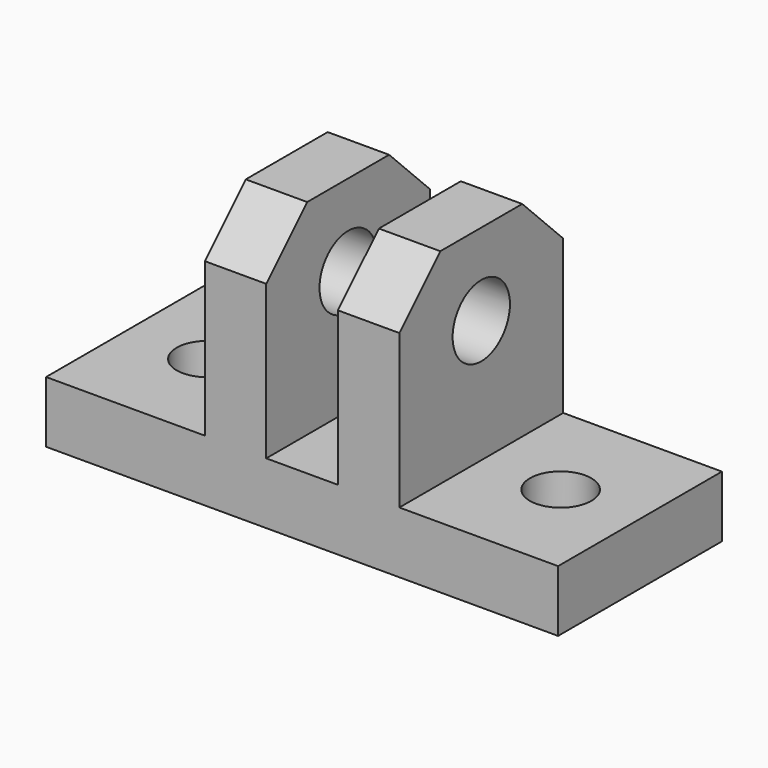
from build123d import *

# Parameters (mm, degrees)
F0_W     = 50
F0_H     = 20
F1_DEPTH = 6
F2_W     = 6
F2_H     = 20
F3_DEPTH = 20
F4_R     = 3.5
F5_DEPTH = 25
F6_SIZE  = 5
F7_R     = 3
F8_DEPTH = 25


# Not quite as in the source:
# - a pattern or mirror of a feature is missing from the dataset's text; its kind, count and spacing are read off the source's solid


with BuildPart() as f1:
    # F0 (on Top) → F1 (new body)
    with BuildSketch(Plane.XY):
        Rectangle(F0_W, F0_H)
    extrude(amount=F1_DEPTH)

    # F2 (on face) → F3 (join)
    with BuildSketch(Plane.XY.offset(6)):
        with Locations((-6.5, 0)):
            Rectangle(F2_W, F2_H)
    f3 = extrude(amount=F3_DEPTH)

    # F3_copies: F3 across plane
    add(f3.mirror(Plane(origin=(0, 0, 0), x_dir=(0, 0, 1), z_dir=(1, 0, 0))))

    # F4 (on face) → F5 (cut)
    with BuildSketch(Plane.YZ.offset(-3.5)):
        with Locations((0, 18)):
            Circle(F4_R)
    f5 = extrude(amount=-F5_DEPTH, mode=Mode.SUBTRACT)

    # F5_copies: F5 across plane
    add(f5.mirror(Plane(origin=(0, 0, 0), x_dir=(0, 0, 1), z_dir=(1, 0, 0))), mode=Mode.SUBTRACT)

    # F6
    f6_edges = [f1.edges().sort_by_distance(p)[0] for p in [
        (-6.5, -10, 26),
        (-6.5, 10, 26),
        (6.5, -10, 26),
        (6.5, 10, 26),
    ]]
    chamfer(f6_edges, length=F6_SIZE)

    # F7 (on face) → F8 (cut)
    with BuildSketch(Plane.XY.offset(6)):
        with Locations((-17.25, 0)):
            Circle(F7_R)
    f8 = extrude(amount=-F8_DEPTH, mode=Mode.SUBTRACT)

    # F8_copies: F8 across plane
    add(f8.mirror(Plane(origin=(0, 0, 0), x_dir=(0, 0, 1), z_dir=(1, 0, 0))), mode=Mode.SUBTRACT)


solid = f1.part
